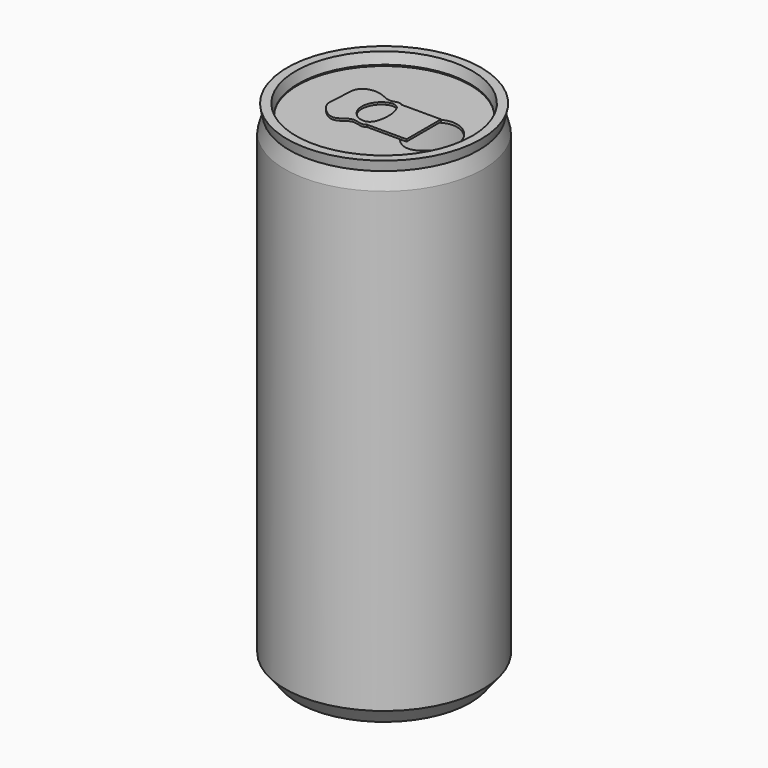
from build123d import *

# Parameters (mm, degrees)
F2_R      = 29.21
F4_R      = 29.21
F0_R      = 25.4
F8_R      = 27.94
F11_R     = 28.575
F13_T     = -2.54
F15_R     = 27.94
F16_DEPTH = 0.762
F18_DEPTH = 0.635


with BuildPart() as f5:
    # F2 (on offset) → F5 section 0
    with BuildSketch(Plane.XY.offset(4.826)):
        Circle(F2_R)
    # F4 (on offset) → F5 section 1
    with BuildSketch(Plane.XY.offset(139.7)):
        Circle(F4_R)
    loft()

    # F0 (on Top) → F6 section 0
    with BuildSketch(Plane.XY):
        Circle(F0_R)
    # F2 (on offset) → F6 section 1
    with BuildSketch(Plane.XY.offset(4.826)):
        Circle(F2_R)
    loft()

    # F4 (on offset) → F9 section 0
    with BuildSketch(Plane.XY.offset(139.7)):
        Circle(F4_R)
    # F8 (on offset) → F9 section 1
    with BuildSketch(Plane.XY.offset(144.272)):
        Circle(F8_R)
    loft()

    # F8 (on offset) → F12 section 0
    with BuildSketch(Plane.XY.offset(144.272)):
        Circle(F8_R)
    # F11 (on offset) → F12 section 1
    with BuildSketch(Plane.XY.offset(147.32)):
        Circle(F11_R)
    loft()

    # F13
    f13_openings = [f5.faces().sort_by_distance(p)[0] for p in [
        (0, 0, 147.32),
    ]]
    offset(amount=F13_T, openings=f13_openings, kind=Kind.INTERSECTION)

    # F15 (on offset) → F16 (join)
    with BuildSketch(Plane.XY.offset(143.764)):
        Circle(F15_R)
        with BuildLine():
            add(Edge.make_bspline(
                [(8.9813927189, -5.08), (10.307283956, -7.660759653), (15.5638091176, -11.3190362963), (24.5819782778, 0.156554303), (16.2046906326, 9.5661078257), (10.4008527308, 7.3320350733), (8.9813927189, 5.08)],
                knots=[0, 0, 0, 0, 0.1793099128, 0.3991725973, 0.6069429862, 0.7863905321, 0.7863905321, 0.7863905321, 0.7863905321], degree=3))
            add(Edge.make_bspline(
                [(8.9813927189, 5.08), (7.2917062072, 2.3992388266), (7.4018764658, -2.0055760179), (8.9813927189, -5.08)],
                knots=[0.7863905321, 0.7863905321, 0.7863905321, 0.7863905321, 1, 1, 1, 1], degree=3))
        make_face(mode=Mode.SUBTRACT)
        with BuildLine():
            add(Edge.make_bspline(
                [(8.9813927189, 5.08), (7.2917062072, 2.3992388266), (7.4018764658, -2.0055760179), (8.9813927189, -5.08)],
                knots=[0.7863905321, 0.7863905321, 0.7863905321, 0.7863905321, 1, 1, 1, 1], degree=3))
            Line((8.9813927189, -5.08), (8.9813927189, 0))
            Line((8.9813927189, 0), (8.9813927189, 5.08))
        make_face()
    extrude(amount=-F16_DEPTH)

    # F17 (on offset) → F18 (join)
    with BuildSketch(Plane.XY.offset(143.764)):
        with BuildLine():
            Line((11.6892714785, -6.35), (11.6892714785, 0))
            Line((11.6892714785, 0), (11.6892714785, 6.35))
            Line((11.6892714785, 6.35), (0, 6.35))
            add(Edge.make_bspline(
                [(0, -6.35), (1.8282559625, -4.4581892492), (1.6638111749, 4.50159086), (0, 6.35)],
                knots=[0.8311304713, 0.8311304713, 0.8311304713, 0.8311304713, 1, 1, 1, 1], degree=3))
            Line((0, -6.35), (11.6892714785, -6.35))
        make_face()
        with BuildLine():
            add(Edge.make_bspline(
                [(0, -6.35), (1.8282559625, -4.4581892492), (1.6638111749, 4.50159086), (0, 6.35)],
                knots=[0.8311304713, 0.8311304713, 0.8311304713, 0.8311304713, 1, 1, 1, 1], degree=3))
            add(Edge.make_bspline(
                [(0, 6.35), (-0.8350152674, 7.2776592654), (-3.4873611567, 5.389008621), (-7.2168226702, 8.4501082119), (-13.9400747086, 7.2984183342), (-13.0107401815, -0.2357314092), (-14.5251656567, -4.4878007238), (-8.0963607859, -10.2798866877), (-4.5226600604, -4.9183886243), (-1.0424695397, -7.4287084101), (0, -6.35)],
                knots=[0, 0, 0, 0, 0.0847503832, 0.1853664744, 0.2931999501, 0.4132443298, 0.5139191398, 0.6328846388, 0.7348412518, 0.8311304713, 0.8311304713, 0.8311304713, 0.8311304713], degree=3))
        make_face()
        with BuildLine():
            add(Edge.make_bspline(
                [(0, 4.6740733087), (-1.0550088408, 5.935167024), (-4.791474758, 5.2358502182), (-7.4773661307, 0.0019184091), (-4.9055168376, -5.0690387184), (1.6043119196, -6.306676079), (1.5736327616, 2.7930479473), (0, 4.6740733087)],
                knots=[0, 0, 0, 0, 0.1740799793, 0.3708117314, 0.5638311353, 0.7403453431, 1, 1, 1, 1], degree=3))
        make_face(mode=Mode.SUBTRACT)
    extrude(amount=F18_DEPTH)


solid = f5.part
